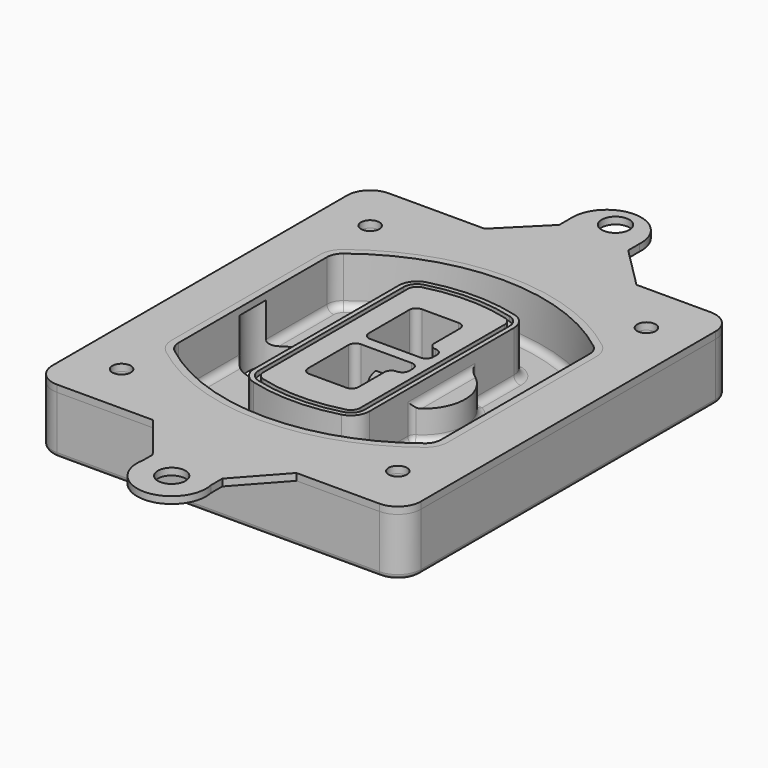
from build123d import *

# Parameters (mm, degrees)
F0_R      = 4
F1_DEPTH  = 25
F2_DEPTH  = 3
F3_DEPTH  = 18
F5_DEPTH  = 21
F6_DEPTH  = 2
F8_DEPTH  = 20
F9_DEPTH  = 16
F10_DEPTH = 25
F7_R      = 6
F7_R_2    = 4
F11_DEPTH = 6
F13_DEPTH = 9
F14_R     = 3
F15_R     = 2
F16_R     = 4
F16_R_2   = 6
F17_DEPTH = 3
F18_DEPTH = 3


# Not quite as in the source:
# - a feature names something its author has since deleted; it is built from what else it names


with BuildPart() as f1:
    # F0 (on Top) → F1 (new body)
    with BuildSketch(Plane.XY):
        with BuildLine():
            ThreePointArc((-80, -80), (-77.0710678119, -87.0710678119), (-70, -90))
            Line((-70, -90), (70, -90))
            ThreePointArc((70, -90), (77.0710678119, -87.0710678119), (80, -80))
            Line((80, -80), (80, 80))
            ThreePointArc((80, 80), (77.0710678119, 87.0710678119), (70, 90))
            Line((70, 90), (-70, 90))
            ThreePointArc((-70, 90), (-77.0710678119, 87.0710678119), (-80, 80))
            Line((-80, 80), (-80, -80))
        make_face()
        with Locations((-60, -67.5)):
            Circle(F0_R, mode=Mode.SUBTRACT)
        with Locations((60, -67.5)):
            Circle(F0_R, mode=Mode.SUBTRACT)
        with Locations((-60, 67.5)):
            Circle(F0_R, mode=Mode.SUBTRACT)
        with BuildLine():
            ThreePointArc((-64, 40.2934422872), (-62.5820384798, 46.4328484224), (-58.6153846154, 51.3286200352))
            ThreePointArc((-58.6153846154, 51.3286200352), (0, 71.5), (58.6153846154, 51.3286200352))
            ThreePointArc((58.6153846154, 51.3286200352), (62.5820384798, 46.4328484224), (64, 40.2934422872))
            Line((64, 40.2934422872), (64, -40.2934422872))
            ThreePointArc((64, -40.2934422872), (62.5820384798, -46.4328484224), (58.6153846154, -51.3286200352))
            ThreePointArc((58.6153846154, -51.3286200352), (0, -71.5), (-58.6153846154, -51.3286200352))
            ThreePointArc((-58.6153846154, -51.3286200352), (-62.5820384798, -46.4328484224), (-64, -40.2934422872))
            Line((-64, -40.2934422872), (-64, 40.2934422872))
        make_face(mode=Mode.SUBTRACT)
        with Locations((60, 67.5)):
            Circle(F0_R, mode=Mode.SUBTRACT)
        with BuildLine():
            ThreePointArc((58.6153846154, 51.3286200352), (0, 71.5), (-58.6153846154, 51.3286200352))
            ThreePointArc((-58.6153846154, 51.3286200352), (-62.5820384798, 46.4328484224), (-64, 40.2934422872))
            Line((-64, 40.2934422872), (-64, -40.2934422872))
            ThreePointArc((-64, -40.2934422872), (-62.5820384798, -46.4328484224), (-58.6153846154, -51.3286200352))
            ThreePointArc((-58.6153846154, -51.3286200352), (0, -71.5), (58.6153846154, -51.3286200352))
            ThreePointArc((58.6153846154, -51.3286200352), (62.5820384798, -46.4328484224), (64, -40.2934422872))
            Line((64, -40.2934422872), (64, 40.2934422872))
            ThreePointArc((64, 40.2934422872), (62.5820384798, 46.4328484224), (58.6153846154, 51.3286200352))
        make_face()
        with BuildLine():
            Line((-60, -40.2934422872), (-60, 40.2934422872))
            ThreePointArc((-60, 40.2934422872), (-58.9871703427, 44.6787323838), (-56.1538461538, 48.1757121072))
            ThreePointArc((-56.1538461538, 48.1757121072), (0, 67.5), (56.1538461538, 48.1757121072))
            ThreePointArc((56.1538461538, 48.1757121072), (58.9871703427, 44.6787323838), (60, 40.2934422872))
            Line((60, 40.2934422872), (60, -40.2934422872))
            ThreePointArc((60, -40.2934422872), (58.9871703427, -44.6787323838), (56.1538461538, -48.1757121072))
            ThreePointArc((56.1538461538, -48.1757121072), (0, -67.5), (-56.1538461538, -48.1757121072))
            ThreePointArc((-56.1538461538, -48.1757121072), (-58.9871703427, -44.6787323838), (-60, -40.2934422872))
        make_face(mode=Mode.SUBTRACT)
        with BuildLine():
            ThreePointArc((-56.1538461538, 48.1757121072), (-58.9871703427, 44.6787323838), (-60, 40.2934422872))
            Line((-60, 40.2934422872), (-60, -40.2934422872))
            ThreePointArc((-60, -40.2934422872), (-58.9871703427, -44.6787323838), (-56.1538461538, -48.1757121072))
            ThreePointArc((-56.1538461538, -48.1757121072), (0, -67.5), (56.1538461538, -48.1757121072))
            ThreePointArc((56.1538461538, -48.1757121072), (58.9871703427, -44.6787323838), (60, -40.2934422872))
            Line((60, -40.2934422872), (60, 40.2934422872))
            ThreePointArc((60, 40.2934422872), (58.9871703427, 44.6787323838), (56.1538461538, 48.1757121072))
            ThreePointArc((56.1538461538, 48.1757121072), (0, 67.5), (-56.1538461538, 48.1757121072))
        make_face()
        with BuildLine():
            ThreePointArc((54.3076923077, 45.8110311612), (56.2910192399, 43.3631453548), (57, 40.2934422872))
            Line((57, 40.2934422872), (57, -40.2934422872))
            ThreePointArc((57, -40.2934422872), (56.2910192399, -43.3631453548), (54.3076923077, -45.8110311612))
            ThreePointArc((54.3076923077, -45.8110311612), (0, -64.5), (-54.3076923077, -45.8110311612))
            ThreePointArc((-54.3076923077, -45.8110311612), (-56.2910192399, -43.3631453548), (-57, -40.2934422872))
            Line((-57, -40.2934422872), (-57, 40.2934422872))
            ThreePointArc((-57, 40.2934422872), (-56.2910192399, 43.3631453548), (-54.3076923077, 45.8110311612))
            ThreePointArc((-54.3076923077, 45.8110311612), (0, 64.5), (54.3076923077, 45.8110311612))
        make_face(mode=Mode.SUBTRACT)
        with BuildLine():
            Line((57, -40.2934422872), (57, 40.2934422872))
            ThreePointArc((57, 40.2934422872), (56.2910192399, 43.3631453548), (54.3076923077, 45.8110311612))
            ThreePointArc((54.3076923077, 45.8110311612), (0, 64.5), (-54.3076923077, 45.8110311612))
            ThreePointArc((-54.3076923077, 45.8110311612), (-56.2910192399, 43.3631453548), (-57, 40.2934422872))
            Line((-57, 40.2934422872), (-57, -40.2934422872))
            ThreePointArc((-57, -40.2934422872), (-56.2910192399, -43.3631453548), (-54.3076923077, -45.8110311612))
            ThreePointArc((-54.3076923077, -45.8110311612), (0, -64.5), (54.3076923077, -45.8110311612))
            ThreePointArc((54.3076923077, -45.8110311612), (56.2910192399, -43.3631453548), (57, -40.2934422872))
        make_face()
    extrude(amount=-F1_DEPTH)

    # F0 (on Top) → F2 (join)
    with BuildSketch(Plane.XY):
        with BuildLine():
            ThreePointArc((-56.1538461538, 48.1757121072), (-58.9871703427, 44.6787323838), (-60, 40.2934422872))
            Line((-60, 40.2934422872), (-60, -40.2934422872))
            ThreePointArc((-60, -40.2934422872), (-58.9871703427, -44.6787323838), (-56.1538461538, -48.1757121072))
            ThreePointArc((-56.1538461538, -48.1757121072), (0, -67.5), (56.1538461538, -48.1757121072))
            ThreePointArc((56.1538461538, -48.1757121072), (58.9871703427, -44.6787323838), (60, -40.2934422872))
            Line((60, -40.2934422872), (60, 40.2934422872))
            ThreePointArc((60, 40.2934422872), (58.9871703427, 44.6787323838), (56.1538461538, 48.1757121072))
            ThreePointArc((56.1538461538, 48.1757121072), (0, 67.5), (-56.1538461538, 48.1757121072))
        make_face()
        with BuildLine():
            ThreePointArc((54.3076923077, 45.8110311612), (56.2910192399, 43.3631453548), (57, 40.2934422872))
            Line((57, 40.2934422872), (57, -40.2934422872))
            ThreePointArc((57, -40.2934422872), (56.2910192399, -43.3631453548), (54.3076923077, -45.8110311612))
            ThreePointArc((54.3076923077, -45.8110311612), (0, -64.5), (-54.3076923077, -45.8110311612))
            ThreePointArc((-54.3076923077, -45.8110311612), (-56.2910192399, -43.3631453548), (-57, -40.2934422872))
            Line((-57, -40.2934422872), (-57, 40.2934422872))
            ThreePointArc((-57, 40.2934422872), (-56.2910192399, 43.3631453548), (-54.3076923077, 45.8110311612))
            ThreePointArc((-54.3076923077, 45.8110311612), (0, 64.5), (54.3076923077, 45.8110311612))
        make_face(mode=Mode.SUBTRACT)
    extrude(amount=F2_DEPTH)

    # F0 (on Top) → F3 (cut)
    with BuildSketch(Plane.XY):
        with BuildLine():
            Line((57, -40.2934422872), (57, 40.2934422872))
            ThreePointArc((57, 40.2934422872), (56.2910192399, 43.3631453548), (54.3076923077, 45.8110311612))
            ThreePointArc((54.3076923077, 45.8110311612), (0, 64.5), (-54.3076923077, 45.8110311612))
            ThreePointArc((-54.3076923077, 45.8110311612), (-56.2910192399, 43.3631453548), (-57, 40.2934422872))
            Line((-57, 40.2934422872), (-57, -40.2934422872))
            ThreePointArc((-57, -40.2934422872), (-56.2910192399, -43.3631453548), (-54.3076923077, -45.8110311612))
            ThreePointArc((-54.3076923077, -45.8110311612), (0, -64.5), (54.3076923077, -45.8110311612))
            ThreePointArc((54.3076923077, -45.8110311612), (56.2910192399, -43.3631453548), (57, -40.2934422872))
        make_face()
    extrude(amount=-F3_DEPTH, mode=Mode.SUBTRACT)

    # F4 (on face) → F5 (join, through all)
    with BuildSketch(Plane.XY.offset(3)):
        with BuildLine():
            ThreePointArc((-25, -39.2465276821), (-23.3511545998, -44.1109737193), (-19.0842911877, -46.9702398883))
            ThreePointArc((-19.0842911877, -46.9702398883), (0, -49.5), (19.0842911877, -46.9702398883))
            ThreePointArc((19.0842911877, -46.9702398883), (23.3511545998, -44.1109737193), (25, -39.2465276821))
            Line((25, -39.2465276821), (25, 39.2465276821))
            ThreePointArc((25, 39.2465276821), (23.3511545998, 44.1109737193), (19.0842911877, 46.9702398883))
            ThreePointArc((19.0842911877, 46.9702398883), (0, 49.5), (-19.0842911877, 46.9702398883))
            ThreePointArc((-19.0842911877, 46.9702398883), (-23.3511545998, 44.1109737193), (-25, 39.2465276821))
            Line((-25, 39.2465276821), (-25, -39.2465276821))
        make_face()
        with BuildLine():
            ThreePointArc((18.5632183908, 45.0393118368), (21.7633659499, 42.89486221), (23, 39.2465276821))
            Line((23, 39.2465276821), (23, -39.2465276821))
            ThreePointArc((23, -39.2465276821), (21.7633659499, -42.89486221), (18.5632183908, -45.0393118368))
            ThreePointArc((18.5632183908, -45.0393118368), (0, -47.5), (-18.5632183908, -45.0393118368))
            ThreePointArc((-18.5632183908, -45.0393118368), (-21.7633659499, -42.89486221), (-23, -39.2465276821))
            Line((-23, -39.2465276821), (-23, 39.2465276821))
            ThreePointArc((-23, 39.2465276821), (-21.7633659499, 42.89486221), (-18.5632183908, 45.0393118368))
            ThreePointArc((-18.5632183908, 45.0393118368), (0, 47.5), (18.5632183908, 45.0393118368))
        make_face(mode=Mode.SUBTRACT)
        with BuildLine():
            Line((23, -39.2465276821), (23, 39.2465276821))
            ThreePointArc((23, 39.2465276821), (21.7633659499, 42.89486221), (18.5632183908, 45.0393118368))
            ThreePointArc((18.5632183908, 45.0393118368), (0, 47.5), (-18.5632183908, 45.0393118368))
            ThreePointArc((-18.5632183908, 45.0393118368), (-21.7633659499, 42.89486221), (-23, 39.2465276821))
            Line((-23, 39.2465276821), (-23, -39.2465276821))
            ThreePointArc((-23, -39.2465276821), (-21.7633659499, -42.89486221), (-18.5632183908, -45.0393118368))
            ThreePointArc((-18.5632183908, -45.0393118368), (0, -47.5), (18.5632183908, -45.0393118368))
            ThreePointArc((18.5632183908, -45.0393118368), (21.7633659499, -42.89486221), (23, -39.2465276821))
        make_face()
        with BuildLine():
            ThreePointArc((18.0421455939, 43.1083837852), (20.1755772999, 41.6787507007), (21, 39.2465276821))
            Line((21, 39.2465276821), (21, -39.2465276821))
            ThreePointArc((21, -39.2465276821), (20.1755772999, -41.6787507007), (18.0421455939, -43.1083837852))
            ThreePointArc((18.0421455939, -43.1083837852), (0, -45.5), (-18.0421455939, -43.1083837852))
            ThreePointArc((-18.0421455939, -43.1083837852), (-20.1755772999, -41.6787507007), (-21, -39.2465276821))
            Line((-21, -39.2465276821), (-21, 39.2465276821))
            ThreePointArc((-21, 39.2465276821), (-20.1755772999, 41.6787507007), (-18.0421455939, 43.1083837852))
            ThreePointArc((-18.0421455939, 43.1083837852), (0, 45.5), (18.0421455939, 43.1083837852))
        make_face(mode=Mode.SUBTRACT)
        with BuildLine():
            Line((21, -39.2465276821), (21, 39.2465276821))
            ThreePointArc((21, 39.2465276821), (20.1755772999, 41.6787507007), (18.0421455939, 43.1083837852))
            ThreePointArc((18.0421455939, 43.1083837852), (0, 45.5), (-18.0421455939, 43.1083837852))
            ThreePointArc((-18.0421455939, 43.1083837852), (-20.1755772999, 41.6787507007), (-21, 39.2465276821))
            Line((-21, 39.2465276821), (-21, -39.2465276821))
            ThreePointArc((-21, -39.2465276821), (-20.1755772999, -41.6787507007), (-18.0421455939, -43.1083837852))
            ThreePointArc((-18.0421455939, -43.1083837852), (0, -45.5), (18.0421455939, -43.1083837852))
            ThreePointArc((18.0421455939, -43.1083837852), (20.1755772999, -41.6787507007), (21, -39.2465276821))
        make_face()
        with BuildLine():
            Line((-8, -2.5), (14, -2.5))
            ThreePointArc((14, -2.5), (16.1213203436, -3.3786796564), (17, -5.5))
            Line((17, -5.5), (17, -7.5))
            ThreePointArc((17, -7.5), (16.1213203436, -9.6213203436), (14, -10.5))
            ThreePointArc((14, -10.5), (11.8786796564, -11.3786796564), (11, -13.5))
            Line((11, -13.5), (11, -27.5))
            ThreePointArc((11, -27.5), (10.1213203436, -29.6213203436), (8, -30.5))
            Line((8, -30.5), (-8, -30.5))
            ThreePointArc((-8, -30.5), (-10.1213203436, -29.6213203436), (-11, -27.5))
            Line((-11, -27.5), (-11, -5.5))
            ThreePointArc((-11, -5.5), (-10.1213203436, -3.3786796564), (-8, -2.5))
        make_face(mode=Mode.SUBTRACT)
        with BuildLine():
            ThreePointArc((-8, 2.5), (-10.1213203436, 3.3786796564), (-11, 5.5))
            Line((-11, 5.5), (-11, 27.5))
            ThreePointArc((-11, 27.5), (-10.1213203436, 29.6213203436), (-8, 30.5))
            Line((-8, 30.5), (8, 30.5))
            ThreePointArc((8, 30.5), (10.1213203436, 29.6213203436), (11, 27.5))
            Line((11, 27.5), (11, 13.5))
            ThreePointArc((11, 13.5), (11.8786796564, 11.3786796564), (14, 10.5))
            ThreePointArc((14, 10.5), (16.1213203436, 9.6213203436), (17, 7.5))
            Line((17, 7.5), (17, 5.5))
            ThreePointArc((17, 5.5), (16.1213203436, 3.3786796564), (14, 2.5))
            Line((14, 2.5), (-8, 2.5))
        make_face(mode=Mode.SUBTRACT)
    extrude(amount=-F5_DEPTH)

    # F4 (on face) → F6 (cut)
    with BuildSketch(Plane.XY.offset(3)):
        with BuildLine():
            Line((23, -39.2465276821), (23, 39.2465276821))
            ThreePointArc((23, 39.2465276821), (21.7633659499, 42.89486221), (18.5632183908, 45.0393118368))
            ThreePointArc((18.5632183908, 45.0393118368), (0, 47.5), (-18.5632183908, 45.0393118368))
            ThreePointArc((-18.5632183908, 45.0393118368), (-21.7633659499, 42.89486221), (-23, 39.2465276821))
            Line((-23, 39.2465276821), (-23, -39.2465276821))
            ThreePointArc((-23, -39.2465276821), (-21.7633659499, -42.89486221), (-18.5632183908, -45.0393118368))
            ThreePointArc((-18.5632183908, -45.0393118368), (0, -47.5), (18.5632183908, -45.0393118368))
            ThreePointArc((18.5632183908, -45.0393118368), (21.7633659499, -42.89486221), (23, -39.2465276821))
        make_face()
        with BuildLine():
            ThreePointArc((18.0421455939, 43.1083837852), (20.1755772999, 41.6787507007), (21, 39.2465276821))
            Line((21, 39.2465276821), (21, -39.2465276821))
            ThreePointArc((21, -39.2465276821), (20.1755772999, -41.6787507007), (18.0421455939, -43.1083837852))
            ThreePointArc((18.0421455939, -43.1083837852), (0, -45.5), (-18.0421455939, -43.1083837852))
            ThreePointArc((-18.0421455939, -43.1083837852), (-20.1755772999, -41.6787507007), (-21, -39.2465276821))
            Line((-21, -39.2465276821), (-21, 39.2465276821))
            ThreePointArc((-21, 39.2465276821), (-20.1755772999, 41.6787507007), (-18.0421455939, 43.1083837852))
            ThreePointArc((-18.0421455939, 43.1083837852), (0, 45.5), (18.0421455939, 43.1083837852))
        make_face(mode=Mode.SUBTRACT)
    extrude(amount=-F6_DEPTH, mode=Mode.SUBTRACT)

    # F7 (on face) → F8 (join)
    with BuildSketch(Plane(origin=(0, 0, -25), x_dir=(1, 0, 0), z_dir=(0, 0, -1))):
        with BuildLine():
            ThreePointArc((3.28842436, 0), (16.7567035675, 13.4682792075), (30.224982775, 0))
            Line((30.224982775, 0), (35.224982775, 0))
            ThreePointArc((35.224982775, 0), (16.7567035675, 18.4682792075), (-1.71157564, 0))
            Line((-1.71157564, 0), (3.28842436, 0))
        make_face()
        with BuildLine():
            Line((3.28842436, 0), (30.224982775, 0))
            ThreePointArc((30.224982775, 0), (16.7567035675, 13.4682792075), (3.28842436, 0))
        make_face()
        with BuildLine():
            ThreePointArc((3.28842436, 0), (16.7567035675, -13.4682792075), (30.224982775, 0))
            Line((30.224982775, 0), (3.28842436, 0))
        make_face()
        with BuildLine():
            Line((35.224982775, 0), (30.224982775, 0))
            ThreePointArc((30.224982775, 0), (16.7567035675, -13.4682792075), (3.28842436, 0))
            Line((3.28842436, 0), (-1.71157564, 0))
            ThreePointArc((-1.71157564, 0), (16.7567035675, -18.4682792075), (35.224982775, 0))
        make_face()
    extrude(amount=-F8_DEPTH)

    # F7 (on face) → F9 (cut)
    with BuildSketch(Plane(origin=(0, 0, -25), x_dir=(1, 0, 0), z_dir=(0, 0, -1))):
        with BuildLine():
            Line((3.28842436, 0), (30.224982775, 0))
            ThreePointArc((30.224982775, 0), (16.7567035675, 13.4682792075), (3.28842436, 0))
        make_face()
        with BuildLine():
            ThreePointArc((3.28842436, 0), (16.7567035675, -13.4682792075), (30.224982775, 0))
            Line((30.224982775, 0), (3.28842436, 0))
        make_face()
    extrude(amount=-F9_DEPTH, mode=Mode.SUBTRACT)

    # F7 (on face) → F10 (cut)
    with BuildSketch(Plane(origin=(0, 0, -25), x_dir=(1, 0, 0), z_dir=(0, 0, -1))):
        with BuildLine():
            Line((-59.0318229325, 0), (-32.0952645175, 0))
            ThreePointArc((-32.0952645175, 0), (-45.563543725, 13.4682792075), (-59.0318229325, 0))
        make_face()
        with BuildLine():
            ThreePointArc((-59.0318229325, 0), (-45.563543725, -13.4682792075), (-32.0952645175, 0))
            Line((-32.0952645175, 0), (-59.0318229325, 0))
        make_face()
    extrude(amount=-F10_DEPTH, mode=Mode.SUBTRACT)

    # F7 (on face) → F11 (cut)
    with BuildSketch(Plane(origin=(0, 0, -25), x_dir=(1, 0, 0), z_dir=(0, 0, -1))):
        with Locations((60, -67.5)):
            Circle(F7_R)
        with Locations((60, -67.5)):
            Circle(F7_R_2, mode=Mode.SUBTRACT)
        with Locations((-60, -67.5)):
            Circle(F7_R)
        with Locations((-60, -67.5)):
            Circle(F7_R_2, mode=Mode.SUBTRACT)
        with Locations((-60, 67.5)):
            Circle(F7_R)
        with Locations((-60, 67.5)):
            Circle(F7_R_2, mode=Mode.SUBTRACT)
        with Locations((60, 67.5)):
            Circle(F7_R)
        with Locations((60, 67.5)):
            Circle(F7_R_2, mode=Mode.SUBTRACT)
    extrude(amount=-F11_DEPTH, mode=Mode.SUBTRACT)

    # F12 (on face) → F13 (cut, through all)
    with BuildSketch(Plane(origin=(0, 0, -9), x_dir=(1, 0, 0), z_dir=(0, 0, -1))):
        with BuildLine():
            Line((11, 13.5), (11, 17.5481537753))
            ThreePointArc((11, 17.5481537753), (2.5696536419, 11.8239143813), (-1.5415842455, 2.5))
            Line((-1.5415842455, 2.5), (3.5224848595, 2.5))
            ThreePointArc((3.5224848595, 2.5), (6.1857188154, 8.3455872281), (11.2536447004, 12.2927168648))
            ThreePointArc((11.2536447004, 12.2927168648), (11.0640958889, 12.8831798879), (11, 13.5))
        make_face()
        with BuildLine():
            ThreePointArc((11.2536447004, -12.2927168648), (6.1857188154, -8.3455872281), (3.5224848595, -2.5))
            Line((3.5224848595, -2.5), (-1.5415842455, -2.5))
            ThreePointArc((-1.5415842455, -2.5), (2.5696536419, -11.8239143813), (11, -17.5481537753))
            Line((11, -17.5481537753), (11, -13.5))
            ThreePointArc((11, -13.5), (11.0640958889, -12.8831798879), (11.2536447004, -12.2927168648))
        make_face()
        with BuildLine():
            ThreePointArc((11.2536447004, 12.2927168648), (6.1857188154, 8.3455872281), (3.5224848595, 2.5))
            Line((3.5224848595, 2.5), (14, 2.5))
            ThreePointArc((14, 2.5), (16.1213203436, 3.3786796564), (17, 5.5))
            Line((17, 5.5), (17, 7.5))
            ThreePointArc((17, 7.5), (16.1213203436, 9.6213203436), (14, 10.5))
            ThreePointArc((14, 10.5), (12.3601599782, 10.9878446101), (11.2536447004, 12.2927168648))
        make_face()
        with BuildLine():
            Line((14, -2.5), (3.5224848595, -2.5))
            ThreePointArc((3.5224848595, -2.5), (6.1857188154, -8.3455872281), (11.2536447004, -12.2927168648))
            ThreePointArc((11.2536447004, -12.2927168648), (12.3601599782, -10.9878446101), (14, -10.5))
            ThreePointArc((14, -10.5), (16.1213203436, -9.6213203436), (17, -7.5))
            Line((17, -7.5), (17, -5.5))
            ThreePointArc((17, -5.5), (16.1213203436, -3.3786796564), (14, -2.5))
        make_face()
    extrude(amount=F13_DEPTH, mode=Mode.SUBTRACT)

    # F14
    f14_edges = [f1.edges().sort_by_distance(p)[0] for p in [
        (-57, -23.703476, -18),
        (-57, 23.703476, -18),
        (25, 0, -5),
        (25, 16.526506, -11.5),
        (25, -16.526506, -11.5),
        (25, -27.886517, -18),
        (35.224983, 0, -18),
        (23.351155, -44.110974, -18),
        (-56.291019, -43.363145, -18),
        (-56.291019, 43.363145, -18),
        (0, 64.5, -18),
        (56.291019, 43.363145, -18),
        (57, 0, -18),
        (56.291019, -43.363145, -18),
        (0, -64.5, -18),
        (-23.351155, 44.110974, -18),
        (0, 49.5, -18),
        (-25, 0, -18),
        (23.351155, 44.110974, -18),
        (-23.351155, -44.110974, -18),
        (25, 27.886517, -18),
        (0, -49.5, -18),
    ]]
    fillet(f14_edges, radius=F14_R)

    # F15
    f15_edges = [f1.edges().sort_by_distance(p)[0] for p in [
        (0, -90, -25),
        (-77.071068, -87.071068, -25),
        (-80, 0, -25),
        (-77.071068, 87.071068, -25),
        (77.071068, -87.071068, -25),
        (0, 90, -25),
        (80, 0, -25),
        (77.071068, 87.071068, -25),
    ]]
    fillet(f15_edges, radius=F15_R)


with BuildPart() as f17:
    # F16 (on face) → F17 (new body, through all)
    with BuildSketch(Plane.XY):
        with BuildLine():
            Line((37.6722225836, 90), (-28.2706206623, 90))
            Line((-28.2706206623, 90), (-70, 90))
            ThreePointArc((-70, 90), (-77.0710678119, 87.0710678119), (-80, 80))
            Line((-80, 80), (-80, -80))
            ThreePointArc((-80, -80), (-77.0710678119, -87.0710678119), (-70, -90))
            Line((-70, -90), (-28.2706206623, -90))
            Line((-28.2706206623, -90), (33.9440070093, -90))
            Line((33.9440070093, -90), (70, -90))
            ThreePointArc((70, -90), (77.0710678119, -87.0710678119), (80, -80))
            Line((80, -80), (80, 80))
            ThreePointArc((80, 80), (77.0710678119, 87.0710678119), (70, 90))
            Line((70, 90), (37.6722225836, 90))
        make_face()
        with Locations((-60, -67.5)):
            Circle(F16_R, mode=Mode.SUBTRACT)
        with Locations((60, -67.5)):
            Circle(F16_R, mode=Mode.SUBTRACT)
        with Locations((-60, 67.5)):
            Circle(F16_R, mode=Mode.SUBTRACT)
        with BuildLine():
            ThreePointArc((-60, 40.2934422872), (-58.9871703427, 44.6787323838), (-56.1538461538, 48.1757121072))
            ThreePointArc((-56.1538461538, 48.1757121072), (0, 67.5), (56.1538461538, 48.1757121072))
            ThreePointArc((56.1538461538, 48.1757121072), (58.9871703427, 44.6787323838), (60, 40.2934422872))
            Line((60, 40.2934422872), (60, -40.2934422872))
            ThreePointArc((60, -40.2934422872), (58.9871703427, -44.6787323838), (56.1538461538, -48.1757121072))
            ThreePointArc((56.1538461538, -48.1757121072), (0, -67.5), (-56.1538461538, -48.1757121072))
            ThreePointArc((-56.1538461538, -48.1757121072), (-58.9871703427, -44.6787323838), (-60, -40.2934422872))
            Line((-60, -40.2934422872), (-60, 40.2934422872))
        make_face(mode=Mode.SUBTRACT)
        with Locations((60, 67.5)):
            Circle(F16_R, mode=Mode.SUBTRACT)
        with BuildLine():
            Line((-10.2706206623, 108), (-28.2706206623, 90))
            Line((-28.2706206623, 90), (37.6722225836, 90))
            Line((37.6722225836, 90), (19.6722225836, 108))
            Line((19.6722225836, 108), (19.6722225836, 114.1535656285))
            ThreePointArc((19.6722225836, 114.1535656285), (4.6583180076, 130.0381981021), (-10.2706206623, 114.0736852805))
            Line((-10.2706206623, 114.0736852805), (-10.2706206623, 108))
        make_face()
        with Locations((4.5791203156, 120)):
            Circle(F16_R_2, mode=Mode.SUBTRACT)
    extrude(amount=F17_DEPTH)

    # F16 (on face) → F18 (join, through all)
    with BuildSketch(Plane.XY):
        with BuildLine():
            Line((33.9440070093, -90), (-28.2706206623, -90))
            Line((-28.2706206623, -90), (-12.484261086, -109.9697484042))
            Line((-12.484261086, -109.9697484042), (-12.484261086, -115.0795741723))
            ThreePointArc((-12.484261086, -115.0795741723), (2.2180253273, -133.0532544208), (16.9203117406, -115.0795741723))
            Line((16.9203117406, -115.0795741723), (16.9203117406, -108.9260085438))
            Line((16.9203117406, -108.9260085438), (33.9440070093, -90))
        make_face()
        with Locations((2.2180253273, -118.0532544208)):
            Circle(F16_R_2, mode=Mode.SUBTRACT)
    extrude(amount=F18_DEPTH)


solid = Compound([f1.part, f17.part])
